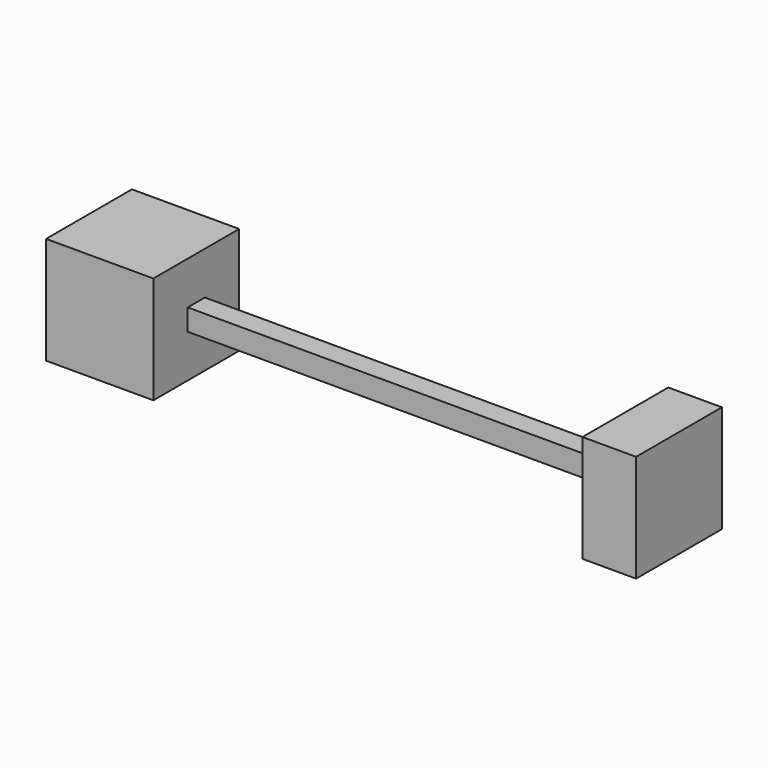
from build123d import *

# Parameters (mm, degrees)
F0_W     = 50
F0_H     = 50
F1_DEPTH = 50
F2_W     = 10
F2_H     = 10
F3_DEPTH = 200
F4_W     = 50
F4_H     = 50
F5_DEPTH = 25


# Not quite as in the source:
# - a feature names something its author has since deleted; it is built from what else it names


with BuildPart() as f1:
    # F0 (on Top) → F1 (new body)
    with BuildSketch(Plane.XY):
        with Locations((25, 25)):
            Rectangle(F0_W, F0_H)
    extrude(amount=F1_DEPTH)

    # F2 (on face) → F3 (join)
    with BuildSketch(Plane.YZ.offset(50)):
        with Locations((25, 25)):
            Rectangle(F2_W, F2_H)
    extrude(amount=F3_DEPTH)

    # F4 (on face) → F5 (join)
    with BuildSketch(Plane.YZ.offset(250)):
        with Locations((25, 25)):
            Rectangle(F4_W, F4_H)
    extrude(amount=F5_DEPTH)


solid = f1.part
